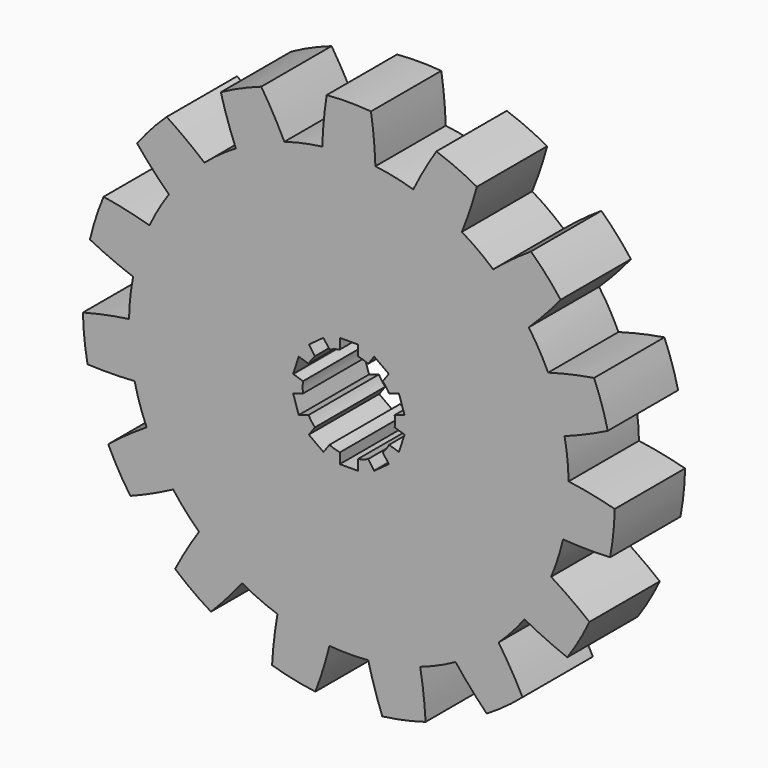
from build123d import *

# Parameters (mm, degrees)
F2_DEPTH = 10
F1_W     = 4.1
F1_H     = 0.2
F3_DEPTH = 10


# Not quite as in the source:
# - a feature of the source that left no trace in its solid (it failed there, or was rolled back) is left out


with BuildPart() as f2:
    # F0 (on Front) → F2 (new body, symmetric)
    with BuildSketch(Plane.XZ):
        with BuildLine():
            ThreePointArc((48.7293634187, -11.2004080646), (49.6813253191, -5.6361258444), (50, 0))
            ThreePointArc((50, 0), (49.9983013941, 0.4121379686), (49.9932056918, 0.8242479348))
            ThreePointArc((49.9932056918, 0.8242479348), (49.7260947684, 5.2264231634), (49.0721049822, 9.587935785))
            ThreePointArc((49.0721049822, 9.587935785), (47.5528258148, 15.4508497187), (45.3358141347, 21.0870566164))
            ThreePointArc((45.3358141347, 21.0870566164), (43.3012701892, 25), (40.9298337882, 28.7184384337))
            ThreePointArc((40.9298337882, 28.7184384337), (37.1572412739, 33.4565303179), (32.8394484508, 37.7037216393))
            ThreePointArc((32.8394484508, 37.7037216393), (29.3892626146, 40.4508497187), (25.7104224964, 42.8832621783))
            ThreePointArc((25.7104224964, 42.8832621783), (20.3368321538, 45.6772728821), (14.6648437927, 47.8010706631))
            ThreePointArc((14.6648437927, 47.8010706631), (10.3955845409, 48.9073800367), (6.0454455831, 49.6331803102))
            ThreePointArc((6.0454455831, 49.6331803102), (0, 50), (-6.0454455831, 49.6331803102))
            ThreePointArc((-6.0454455831, 49.6331803102), (-10.3955845409, 48.9073800367), (-14.6648437927, 47.8010706631))
            ThreePointArc((-14.6648437927, 47.8010706631), (-20.3368321538, 45.6772728821), (-25.7104224964, 42.8832621783))
            ThreePointArc((-25.7104224964, 42.8832621783), (-29.3892626146, 40.4508497187), (-32.8394484508, 37.7037216393))
            ThreePointArc((-32.8394484508, 37.7037216393), (-37.1572412739, 33.4565303179), (-40.9298337882, 28.7184384337))
            ThreePointArc((-40.9298337882, 28.7184384337), (-43.3012701892, 25), (-45.3358141347, 21.0870566164))
            ThreePointArc((-45.3358141347, 21.0870566164), (-47.5528258148, 15.4508497187), (-49.0721049822, 9.587935785))
            ThreePointArc((-49.0721049822, 9.587935785), (-49.7260947684, 5.2264231634), (-49.9932056918, 0.8242479348))
            ThreePointArc((-49.9932056918, 0.8242479348), (-49.7260947684, -5.2264231634), (-48.7293634187, -11.2004080646))
            ThreePointArc((-48.7293634187, -11.2004080646), (-47.5528258148, -15.4508497187), (-46.0063178108, -19.5810807029))
            ThreePointArc((-46.0063178108, -19.5810807029), (-43.3012701892, -25), (-39.9608722277, -30.0520996073))
            ThreePointArc((-39.9608722277, -30.0520996073), (-37.1572412739, -33.4565303179), (-34.064519626, -36.6006625985))
            ThreePointArc((-34.064519626, -36.6006625985), (-29.3892626146, -40.4508497187), (-24.2827831954, -43.7075101131))
            ThreePointArc((-24.2827831954, -43.7075101131), (-20.3368321538, -45.6772728821), (-16.2326565314, -47.2916574242))
            ThreePointArc((-16.2326565314, -47.2916574242), (-10.3955845409, -48.9073800367), (-4.4059803465, -49.8054950501))
            ThreePointArc((-4.4059803465, -49.8054950501), (0, -50), (4.4059803465, -49.8054950501))
            ThreePointArc((4.4059803465, -49.8054950501), (10.3955845409, -48.9073800367), (16.2326565314, -47.2916574242))
            ThreePointArc((16.2326565314, -47.2916574242), (20.3368321538, -45.6772728821), (24.2827831954, -43.7075101131))
            ThreePointArc((24.2827831954, -43.7075101131), (29.3892626146, -40.4508497187), (34.064519626, -36.6006625985))
            ThreePointArc((34.064519626, -36.6006625985), (37.1572412739, -33.4565303179), (39.9608722277, -30.0520996073))
            ThreePointArc((39.9608722277, -30.0520996073), (43.3012701892, -25), (46.0063178108, -19.5810807029))
            ThreePointArc((46.0063178108, -19.5810807029), (47.5528258148, -15.4508497187), (48.7293634187, -11.2004080646))
        make_face()
        with BuildLine():
            ThreePointArc((49.9932056918, 0.8242479348), (49.9983013941, 0.4121379686), (50, 0))
            ThreePointArc((50, 0), (49.6813253191, -5.6361258444), (48.7293634187, -11.2004080646))
            ThreePointArc((48.7293634187, -11.2004080646), (54.0795856679, -11.4153231348), (59.433119675, -11.3116880129))
            ThreePointArc((59.433119675, -11.3116880129), (60.1685746698, -6.3239720277), (60.486195595, -1.2923399121))
            ThreePointArc((60.486195595, -1.2923399121), (55.2711961039, -0.077907159), (49.9932056918, 0.8242479348))
        make_face()
        with BuildLine():
            ThreePointArc((45.3358141347, 21.0870566164), (47.5528258148, 15.4508497187), (49.0721049822, 9.587935785))
            ThreePointArc((49.0721049822, 9.587935785), (54.0471900496, 11.5677325362), (58.8957345225, 13.8398863816))
            ThreePointArc((58.8957345225, 13.8398863816), (57.5389192359, 18.6955281597), (55.7825312334, 23.4213408923))
            ThreePointArc((55.7825312334, 23.4213408923), (50.5244378355, 22.4096490308), (45.3358141347, 21.0870566164))
        make_face()
        with BuildLine():
            ThreePointArc((54.7312472383, -25.7825634052), (50.4610624428, -22.5519924933), (46.0063178108, -19.5810807029))
            ThreePointArc((46.0063178108, -19.5810807029), (43.3012701892, -25), (39.9608722277, -30.0520996073))
            ThreePointArc((39.9608722277, -30.0520996073), (44.7611296266, -32.4245657308), (49.6939785027, -34.5073687866))
            ThreePointArc((49.6939785027, -34.5073687866), (52.394536929, -30.25), (54.7312472383, -25.7825634052))
        make_face()
        with BuildLine():
            ThreePointArc((32.8394484508, 37.7037216393), (37.1572412739, 33.4565303179), (40.9298337882, 28.7184384337))
            ThreePointArc((40.9298337882, 28.7184384337), (44.6695442683, 32.5506221621), (48.1747418201, 36.5984186894))
            ThreePointArc((48.1747418201, 36.5984186894), (44.9602619414, 40.4824016847), (41.4335604532, 44.0852590802))
            ThreePointArc((41.4335604532, 44.0852590802), (37.0415452653, 41.022373318), (32.8394484508, 37.7037216393))
        make_face()
        with BuildLine():
            ThreePointArc((39.5127690163, -45.8147474582), (36.9257526611, -41.1266334471), (34.064519626, -36.6006625985))
            ThreePointArc((34.064519626, -36.6006625985), (29.3892626146, -40.4508497187), (24.2827831954, -43.7075101131))
            ThreePointArc((24.2827831954, -43.7075101131), (27.7030676308, -47.827306344), (31.3622969917, -51.7364120075))
            ThreePointArc((31.3622969917, -51.7364120075), (35.5610077637, -48.9455281597), (39.5127690164, -45.8147474582))
        make_face()
        with BuildLine():
            ThreePointArc((14.6648437927, 47.8010706631), (20.3368321538, 45.6772728821), (25.7104224964, 42.8832621783))
            ThreePointArc((25.7104224964, 42.8832621783), (27.5681284731, 47.905213503), (29.1238986033, 53.0287519196))
            ThreePointArc((29.1238986033, 53.0287519196), (24.6075669061, 55.2695001874), (19.9203506586, 57.1264354711))
            ThreePointArc((19.9203506586, 57.1264354711), (17.1538330068, 52.5419565819), (14.6648437927, 47.8010706631))
        make_face()
        with BuildLine():
            ThreePointArc((17.4621740692, -57.9251454618), (17.0056447843, -52.5901058542), (16.2326565314, -47.2916574242))
            ThreePointArc((16.2326565314, -47.2916574242), (10.3955845409, -48.9073800367), (4.4059803465, -49.8054950501))
            ThreePointArc((4.4059803465, -49.8054950501), (5.8548935672, -54.9602711929), (7.6077894133, -60.0197595817))
            ThreePointArc((7.6077894133, -60.0197595817), (12.5786572945, -59.1779298444), (17.4621740692, -57.9251454618))
        make_face()
        with BuildLine():
            ThreePointArc((-6.0454455831, 49.6331803102), (0, 50), (6.0454455831, 49.6331803102))
            ThreePointArc((6.0454455831, 49.6331803102), (5.6999328162, 54.9765582241), (5.0372687356, 60.2899321917))
            ThreePointArc((5.0372687356, 60.2899321917), (0, 60.5), (-5.0372687356, 60.2899321917))
            ThreePointArc((-5.0372687356, 60.2899321917), (-5.6999328162, 54.9765582241), (-6.0454455831, 49.6331803102))
        make_face()
        with BuildLine():
            ThreePointArc((-7.6077894133, -60.0197595817), (-5.8548935672, -54.9602711929), (-4.4059803465, -49.8054950501))
            ThreePointArc((-4.4059803465, -49.8054950501), (-10.3955845409, -48.9073800367), (-16.2326565314, -47.2916574242))
            ThreePointArc((-16.2326565314, -47.2916574242), (-17.0056447843, -52.5901058542), (-17.4621740692, -57.9251454618))
            ThreePointArc((-17.4621740692, -57.9251454618), (-12.5786572945, -59.1779298444), (-7.6077894133, -60.0197595817))
        make_face()
        with BuildLine():
            ThreePointArc((-25.7104224964, 42.8832621783), (-20.3368321538, 45.6772728821), (-14.6648437927, 47.8010706631))
            ThreePointArc((-14.6648437927, 47.8010706631), (-17.1538330068, 52.5419565819), (-19.9203506586, 57.1264354711))
            ThreePointArc((-19.9203506586, 57.1264354711), (-24.6075669061, 55.2695001874), (-29.1238986033, 53.0287519196))
            ThreePointArc((-29.1238986033, 53.0287519196), (-27.5681284731, 47.905213503), (-25.7104224964, 42.8832621783))
        make_face()
        with BuildLine():
            ThreePointArc((-31.3622969917, -51.7364120075), (-27.7030676308, -47.827306344), (-24.2827831954, -43.7075101131))
            ThreePointArc((-24.2827831954, -43.7075101131), (-29.3892626146, -40.4508497187), (-34.064519626, -36.6006625985))
            ThreePointArc((-34.064519626, -36.6006625985), (-36.9257526611, -41.1266334471), (-39.5127690164, -45.8147474582))
            ThreePointArc((-39.5127690163, -45.8147474582), (-35.5610077637, -48.9455281597), (-31.3622969917, -51.7364120075))
        make_face()
        with BuildLine():
            ThreePointArc((-40.9298337882, 28.7184384337), (-37.1572412739, 33.4565303179), (-32.8394484508, 37.7037216393))
            ThreePointArc((-32.8394484508, 37.7037216393), (-37.0415452653, 41.022373318), (-41.4335604532, 44.0852590802))
            ThreePointArc((-41.4335604532, 44.0852590802), (-44.9602619414, 40.4824016847), (-48.1747418201, 36.5984186894))
            ThreePointArc((-48.1747418201, 36.5984186894), (-44.6695442683, 32.5506221621), (-40.9298337882, 28.7184384337))
        make_face()
        with BuildLine():
            ThreePointArc((-49.6939785027, -34.5073687866), (-44.7611296266, -32.4245657308), (-39.9608722277, -30.0520996073))
            ThreePointArc((-39.9608722277, -30.0520996073), (-43.3012701892, -25), (-46.0063178108, -19.5810807029))
            ThreePointArc((-46.0063178108, -19.5810807029), (-50.4610624428, -22.5519924933), (-54.7312472383, -25.7825634052))
            ThreePointArc((-54.7312472383, -25.7825634052), (-52.394536929, -30.25), (-49.6939785027, -34.5073687866))
        make_face()
        with BuildLine():
            ThreePointArc((-49.0721049822, 9.587935785), (-47.5528258148, 15.4508497187), (-45.3358141347, 21.0870566164))
            ThreePointArc((-45.3358141347, 21.0870566164), (-50.5244378355, 22.4096490308), (-55.7825312334, 23.4213408923))
            ThreePointArc((-55.7825312334, 23.4213408923), (-57.5389192359, 18.6955281597), (-58.8957345225, 13.8398863816))
            ThreePointArc((-58.8957345225, 13.8398863816), (-54.0471900496, 11.5677325362), (-49.0721049822, 9.587935785))
        make_face()
        with BuildLine():
            ThreePointArc((-59.433119675, -11.3116880129), (-54.0795856679, -11.4153231348), (-48.7293634187, -11.2004080646))
            ThreePointArc((-48.7293634187, -11.2004080646), (-49.7260947684, -5.2264231634), (-49.9932056918, 0.8242479348))
            ThreePointArc((-49.9932056918, 0.8242479348), (-55.2711961039, -0.077907159), (-60.486195595, -1.2923399121))
            ThreePointArc((-60.486195595, -1.2923399121), (-60.1685746698, -6.3239720277), (-59.433119675, -11.3116880129))
        make_face()
    extrude(amount=F2_DEPTH, both=True)

    # F1 (on Front) → F3 (cut, symmetric)
    with BuildSketch(Plane.XZ):
        with BuildLine():
            ThreePointArc((10.4274046286, -1.2325715847), (10.4818354452, -0.6173537882), (10.5, 0))
            ThreePointArc((10.5, 0), (10.4818354452, 0.6173537882), (10.4274046286, 1.2325715847))
            Line((10.4274046286, 1.2325715847), (6.6339393539, 0))
            Line((6.6339393539, 0), (10.4274046286, -1.2325715847))
        make_face()
        with BuildLine():
            Line((6.6339393539, 0), (10.4274046286, 1.2325715847))
            ThreePointArc((10.4274046286, 1.2325715847), (9.9860934211, 3.2446784409), (9.1604349517, 5.1319033015))
            Line((9.1604349517, 5.1319033015), (5.3669696769, 3.8993317168))
            Line((5.3669696769, 3.8993317168), (3.3169696769, 1.0777487798))
            Line((3.3169696769, 1.0777487798), (6.6339393539, 0))
        make_face()
        with BuildLine():
            ThreePointArc((9.1604349517, 5.1319033015), (9.9860934211, 3.2446784409), (10.4274046286, 1.2325715847))
            Line((10.4274046286, 1.2325715847), (12.4741384663, 1.8975957216))
            Line((12.4741384663, 1.8975957216), (12.6643497696, 1.9593991204))
            Line((12.6643497696, 1.9593991204), (11.3973800927, 5.8587308372))
            Line((11.3973800927, 5.8587308372), (11.2071687894, 5.7969274384))
            Line((11.2071687894, 5.7969274384), (9.1604349517, 5.1319033015))
        make_face()
        with BuildLine():
            Line((12.4741384663, -1.8975957216), (10.4274046286, -1.2325715847))
            ThreePointArc((10.4274046286, -1.2325715847), (9.9860934211, -3.2446784409), (9.1604349517, -5.1319033015))
            Line((9.1604349517, -5.1319033015), (11.2071687894, -5.7969274384))
            Line((11.2071687894, -5.7969274384), (11.3973800927, -5.8587308372))
            Line((11.3973800927, -5.8587308372), (12.6643497696, -1.9593991204))
            Line((12.6643497696, -1.9593991204), (12.4741384663, -1.8975957216))
        make_face()
        with BuildLine():
            ThreePointArc((9.1604349517, -5.1319033015), (9.9860934211, -3.2446784409), (10.4274046286, -1.2325715847))
            Line((10.4274046286, -1.2325715847), (6.6339393539, 0))
            Line((6.6339393539, 0), (3.3169696769, -1.0777487798))
            Line((3.3169696769, -1.0777487798), (5.3669696769, -3.8993317168))
            Line((5.3669696769, -3.8993317168), (9.1604349517, -5.1319033015))
        make_face()
        with BuildLine():
            Line((5.3669696769, 3.8993317168), (9.1604349517, 5.1319033015))
            ThreePointArc((9.1604349517, 5.1319033015), (8.4946784409, 6.1717451491), (7.7114601519, 7.1262460192))
            Line((7.7114601519, 7.1262460192), (5.3669696769, 3.8993317168))
        make_face()
        Polygon((3.3169696769, -1.0777487798), (6.6339393539, 0), (3.3169696769, 1.0777487798), (2.5339393539, 0), align=None)
        with BuildLine():
            ThreePointArc((7.7114601519, -7.1262460192), (8.4946784409, -6.1717451491), (9.1604349517, -5.1319033015))
            Line((9.1604349517, -5.1319033015), (5.3669696769, -3.8993317168))
            Line((5.3669696769, -3.8993317168), (7.7114601519, -7.1262460192))
        make_face()
        with BuildLine():
            Line((5.3669696769, 3.8993317168), (7.7114601519, 7.1262460192))
            ThreePointArc((7.7114601519, 7.1262460192), (6.1717451491, 8.4946784409), (4.3944904749, 9.5361655536))
            Line((4.3944904749, 9.5361655536), (2.05, 6.3092512512))
            Line((2.05, 6.3092512512), (2.05, 2.821582937))
            Line((2.05, 2.821582937), (5.3669696769, 3.8993317168))
        make_face()
        with BuildLine():
            ThreePointArc((4.3944904749, 9.5361655536), (6.1717451491, 8.4946784409), (7.7114601519, 7.1262460192))
            Line((7.7114601519, 7.1262460192), (8.9764112295, 8.8673018128))
            Line((8.9764112295, 8.8673018128), (9.09396828, 9.0291052116))
            Line((9.09396828, 9.0291052116), (5.776998603, 11.439024746))
            Line((5.776998603, 11.439024746), (5.6594415526, 11.2772213472))
            Line((5.6594415526, 11.2772213472), (4.3944904749, 9.5361655536))
        make_face()
        Polygon((3.3169696769, 1.0777487798), (5.3669696769, 3.8993317168), (2.05, 2.821582937), (2.05, 1.4894121824), align=None)
        Polygon((2.5339393539, 0), (3.3169696769, 1.0777487798), (2.05, 1.4894121824), (2.05, 0.6660853773), align=None)
        Polygon((2.05, -1.4894121824), (3.3169696769, -1.0777487798), (2.5339393539, 0), (2.05, -0.6660853773), align=None)
        Polygon((5.3669696769, -3.8993317168), (3.3169696769, -1.0777487798), (2.05, -1.4894121824), (2.05, -2.821582937), align=None)
        with BuildLine():
            Line((8.9764112295, -8.8673018128), (7.7114601519, -7.1262460192))
            ThreePointArc((7.7114601519, -7.1262460192), (6.1717451491, -8.4946784409), (4.3944904749, -9.5361655536))
            Line((4.3944904749, -9.5361655536), (5.6594415526, -11.2772213472))
            Line((5.6594415526, -11.2772213472), (5.776998603, -11.439024746))
            Line((5.776998603, -11.439024746), (9.09396828, -9.0291052116))
            Line((9.09396828, -9.0291052116), (8.9764112295, -8.8673018128))
        make_face()
        with BuildLine():
            ThreePointArc((4.3944904749, -9.5361655536), (6.1717451491, -8.4946784409), (7.7114601519, -7.1262460192))
            Line((7.7114601519, -7.1262460192), (5.3669696769, -3.8993317168))
            Line((5.3669696769, -3.8993317168), (2.05, -2.821582937))
            Line((2.05, -2.821582937), (2.05, -6.3092512512))
            Line((2.05, -6.3092512512), (4.3944904749, -9.5361655536))
        make_face()
        with BuildLine():
            Line((2.05, 6.3092512512), (4.3944904749, 9.5361655536))
            ThreePointArc((4.3944904749, 9.5361655536), (3.2446784409, 9.9860934211), (2.05, 10.2979366865))
            Line((2.05, 10.2979366865), (2.05, 6.3092512512))
        make_face()
        Polygon((0.7830303231, 2.4099195344), (2.05, 2.821582937), (2.05, 6.3092512512), (0, 3.4876683142), align=None)
        Polygon((2.05, 1.4894121824), (2.05, 2.821582937), (0.7830303231, 2.4099195344), (1.2669696769, 1.7438341571), align=None)
        Polygon((2.05, 0.6660853773), (2.05, 1.4894121824), (1.2669696769, 1.7438341571), align=None)
        Polygon((2.05, -0.6660853773), (2.5339393539, 0), (2.05, 0.6660853773), align=None)
        Polygon((1.2669696769, -1.7438341571), (2.05, -1.4894121824), (2.05, -0.6660853773), align=None)
        Polygon((2.05, -2.821582937), (2.05, -1.4894121824), (1.2669696769, -1.7438341571), (0.7830303231, -2.4099195344), align=None)
        with BuildLine():
            ThreePointArc((2.05, -10.2979366865), (3.2446784409, -9.9860934211), (4.3944904749, -9.5361655536))
            Line((4.3944904749, -9.5361655536), (2.05, -6.3092512512))
            Line((2.05, -6.3092512512), (2.05, -10.2979366865))
        make_face()
        Polygon((2.05, -6.3092512512), (2.05, -2.821582937), (0.7830303231, -2.4099195344), (0, -3.4876683142), align=None)
        with BuildLine():
            Line((2.05, 6.3092512512), (2.05, 10.2979366865))
            ThreePointArc((2.05, 10.2979366865), (0, 10.5), (-2.05, 10.2979366865))
            Line((-2.05, 10.2979366865), (-2.05, 6.3092512512))
            Line((-2.05, 6.3092512512), (0, 3.4876683142))
            Line((0, 3.4876683142), (2.05, 6.3092512512))
        make_face()
        with BuildLine():
            ThreePointArc((-2.05, 10.2979366865), (0, 10.5), (2.05, 10.2979366865))
            Line((2.05, 10.2979366865), (2.05, 12.45))
            Line((2.05, 12.45), (2.05, 12.65))
            Line((2.05, 12.65), (-2.05, 12.65))
            Line((-2.05, 12.65), (-2.05, 12.45))
            Line((-2.05, 12.45), (-2.05, 10.2979366865))
        make_face()
        Polygon((0, 2.1554975597), (0.7830303231, 2.4099195344), (0, 3.4876683142), (-0.7830303231, 2.4099195344), align=None)
        Polygon((1.2669696769, 1.7438341571), (0.7830303231, 2.4099195344), (0, 2.1554975597), align=None)
        Polygon((2.05, -0.6660853773), (2.05, 0.6660853773), (1.2669696769, 1.7438341571), (0, 2.1554975597), (-1.2669696769, 1.7438341571), (-2.05, 0.6660853773), (-2.05, -0.6660853773), (-1.2669696769, -1.7438341571), (0, -2.1554975597), (1.2669696769, -1.7438341571), align=None)
        Polygon((0.7830303231, -2.4099195344), (1.2669696769, -1.7438341571), (0, -2.1554975597), align=None)
        with BuildLine():
            Line((2.05, -12.45), (2.05, -10.2979366865))
            ThreePointArc((2.05, -10.2979366865), (0, -10.5), (-2.05, -10.2979366865))
            Line((-2.05, -10.2979366865), (-2.05, -12.45))
            Line((-2.05, -12.45), (2.05, -12.45))
        make_face()
        with BuildLine():
            ThreePointArc((-2.05, -10.2979366865), (0, -10.5), (2.05, -10.2979366865))
            Line((2.05, -10.2979366865), (2.05, -6.3092512512))
            Line((2.05, -6.3092512512), (0, -3.4876683142))
            Line((0, -3.4876683142), (-2.05, -6.3092512512))
            Line((-2.05, -6.3092512512), (-2.05, -10.2979366865))
        make_face()
        Polygon((0, -3.4876683142), (0.7830303231, -2.4099195344), (0, -2.1554975597), (-0.7830303231, -2.4099195344), align=None)
        with BuildLine():
            Line((-2.05, 6.3092512512), (-2.05, 10.2979366865))
            ThreePointArc((-2.05, 10.2979366865), (-3.2446784409, 9.9860934211), (-4.3944904749, 9.5361655536))
            Line((-4.3944904749, 9.5361655536), (-2.05, 6.3092512512))
        make_face()
        Polygon((-0.7830303231, 2.4099195344), (0, 3.4876683142), (-2.05, 6.3092512512), (-2.05, 2.821582937), align=None)
        Polygon((-1.2669696769, 1.7438341571), (0, 2.1554975597), (-0.7830303231, 2.4099195344), align=None)
        Polygon((-0.7830303231, -2.4099195344), (0, -2.1554975597), (-1.2669696769, -1.7438341571), align=None)
        with BuildLine():
            ThreePointArc((-4.3944904749, -9.5361655536), (-3.2446784409, -9.9860934211), (-2.05, -10.2979366865))
            Line((-2.05, -10.2979366865), (-2.05, -6.3092512512))
            Line((-2.05, -6.3092512512), (-4.3944904749, -9.5361655536))
        make_face()
        with Locations((0, -12.55)):
            Rectangle(F1_W, F1_H)
        Polygon((-2.05, -6.3092512512), (0, -3.4876683142), (-0.7830303231, -2.4099195344), (-2.05, -2.821582937), align=None)
        with BuildLine():
            Line((-2.05, 6.3092512512), (-4.3944904749, 9.5361655536))
            ThreePointArc((-4.3944904749, 9.5361655536), (-6.1717451491, 8.4946784409), (-7.7114601519, 7.1262460192))
            Line((-7.7114601519, 7.1262460192), (-5.3669696769, 3.8993317168))
            Line((-5.3669696769, 3.8993317168), (-2.05, 2.821582937))
            Line((-2.05, 2.821582937), (-2.05, 6.3092512512))
        make_face()
        with BuildLine():
            ThreePointArc((-7.7114601519, 7.1262460192), (-6.1717451491, 8.4946784409), (-4.3944904749, 9.5361655536))
            Line((-4.3944904749, 9.5361655536), (-5.6594415526, 11.2772213472))
            Line((-5.6594415526, 11.2772213472), (-5.776998603, 11.439024746))
            Line((-5.776998603, 11.439024746), (-9.09396828, 9.0291052116))
            Line((-9.09396828, 9.0291052116), (-8.9764112295, 8.8673018128))
            Line((-8.9764112295, 8.8673018128), (-7.7114601519, 7.1262460192))
        make_face()
        Polygon((-1.2669696769, 1.7438341571), (-0.7830303231, 2.4099195344), (-2.05, 2.821582937), (-2.05, 1.4894121824), align=None)
        Polygon((-2.05, 0.6660853773), (-1.2669696769, 1.7438341571), (-2.05, 1.4894121824), align=None)
        Polygon((-2.05, -1.4894121824), (-1.2669696769, -1.7438341571), (-2.05, -0.6660853773), align=None)
        Polygon((-0.7830303231, -2.4099195344), (-1.2669696769, -1.7438341571), (-2.05, -1.4894121824), (-2.05, -2.821582937), align=None)
        with BuildLine():
            Line((-5.6594415526, -11.2772213472), (-4.3944904749, -9.5361655536))
            ThreePointArc((-4.3944904749, -9.5361655536), (-6.1717451491, -8.4946784409), (-7.7114601519, -7.1262460192))
            Line((-7.7114601519, -7.1262460192), (-8.9764112295, -8.8673018128))
            Line((-8.9764112295, -8.8673018128), (-9.09396828, -9.0291052116))
            Line((-9.09396828, -9.0291052116), (-5.776998603, -11.439024746))
            Line((-5.776998603, -11.439024746), (-5.6594415526, -11.2772213472))
        make_face()
        with BuildLine():
            ThreePointArc((-7.7114601519, -7.1262460192), (-6.1717451491, -8.4946784409), (-4.3944904749, -9.5361655536))
            Line((-4.3944904749, -9.5361655536), (-2.05, -6.3092512512))
            Line((-2.05, -6.3092512512), (-2.05, -2.821582937))
            Line((-2.05, -2.821582937), (-5.3669696769, -3.8993317168))
            Line((-5.3669696769, -3.8993317168), (-7.7114601519, -7.1262460192))
        make_face()
        with BuildLine():
            Line((-5.3669696769, 3.8993317168), (-7.7114601519, 7.1262460192))
            ThreePointArc((-7.7114601519, 7.1262460192), (-8.4946784409, 6.1717451491), (-9.1604349517, 5.1319033015))
            Line((-9.1604349517, 5.1319033015), (-5.3669696769, 3.8993317168))
        make_face()
        Polygon((-2.05, 1.4894121824), (-2.05, 2.821582937), (-5.3669696769, 3.8993317168), (-3.3169696769, 1.0777487798), align=None)
        Polygon((-2.05, 0.6660853773), (-2.05, 1.4894121824), (-3.3169696769, 1.0777487798), (-2.5339393539, 0), align=None)
        Polygon((-2.05, -0.6660853773), (-2.05, 0.6660853773), (-2.5339393539, 0), align=None)
        Polygon((-2.05, -1.4894121824), (-2.05, -0.6660853773), (-2.5339393539, 0), (-3.3169696769, -1.0777487798), align=None)
        Polygon((-2.05, -2.821582937), (-2.05, -1.4894121824), (-3.3169696769, -1.0777487798), (-5.3669696769, -3.8993317168), align=None)
        with BuildLine():
            ThreePointArc((-9.1604349517, -5.1319033015), (-8.4946784409, -6.1717451491), (-7.7114601519, -7.1262460192))
            Line((-7.7114601519, -7.1262460192), (-5.3669696769, -3.8993317168))
            Line((-5.3669696769, -3.8993317168), (-9.1604349517, -5.1319033015))
        make_face()
        with BuildLine():
            Line((-5.3669696769, 3.8993317168), (-9.1604349517, 5.1319033015))
            ThreePointArc((-9.1604349517, 5.1319033015), (-9.9860934211, 3.2446784409), (-10.4274046286, 1.2325715847))
            Line((-10.4274046286, 1.2325715847), (-6.6339393539, 0))
            Line((-6.6339393539, 0), (-3.3169696769, 1.0777487798))
            Line((-3.3169696769, 1.0777487798), (-5.3669696769, 3.8993317168))
        make_face()
        with BuildLine():
            ThreePointArc((-10.4274046286, 1.2325715847), (-9.9860934211, 3.2446784409), (-9.1604349517, 5.1319033015))
            Line((-9.1604349517, 5.1319033015), (-11.2071687894, 5.7969274384))
            Line((-11.2071687894, 5.7969274384), (-11.3973800927, 5.8587308372))
            Line((-11.3973800927, 5.8587308372), (-12.6643497696, 1.9593991204))
            Line((-12.6643497696, 1.9593991204), (-12.4741384663, 1.8975957216))
            Line((-12.4741384663, 1.8975957216), (-10.4274046286, 1.2325715847))
        make_face()
        Polygon((-2.5339393539, 0), (-3.3169696769, 1.0777487798), (-6.6339393539, 0), (-3.3169696769, -1.0777487798), align=None)
        with BuildLine():
            Line((-5.3669696769, -3.8993317168), (-3.3169696769, -1.0777487798))
            Line((-3.3169696769, -1.0777487798), (-6.6339393539, 0))
            Line((-6.6339393539, 0), (-10.4274046286, -1.2325715847))
            ThreePointArc((-10.4274046286, -1.2325715847), (-9.9860934211, -3.2446784409), (-9.1604349517, -5.1319033015))
            Line((-9.1604349517, -5.1319033015), (-5.3669696769, -3.8993317168))
        make_face()
        with BuildLine():
            Line((-11.2071687894, -5.7969274384), (-9.1604349517, -5.1319033015))
            ThreePointArc((-9.1604349517, -5.1319033015), (-9.9860934211, -3.2446784409), (-10.4274046286, -1.2325715847))
            Line((-10.4274046286, -1.2325715847), (-12.4741384663, -1.8975957216))
            Line((-12.4741384663, -1.8975957216), (-12.6643497696, -1.9593991204))
            Line((-12.6643497696, -1.9593991204), (-11.3973800927, -5.8587308372))
            Line((-11.3973800927, -5.8587308372), (-11.2071687894, -5.7969274384))
        make_face()
        with BuildLine():
            Line((-6.6339393539, 0), (-10.4274046286, 1.2325715847))
            ThreePointArc((-10.4274046286, 1.2325715847), (-10.5, 0), (-10.4274046286, -1.2325715847))
            Line((-10.4274046286, -1.2325715847), (-6.6339393539, 0))
        make_face()
    extrude(amount=F3_DEPTH, both=True, mode=Mode.SUBTRACT)


solid = f2.part
